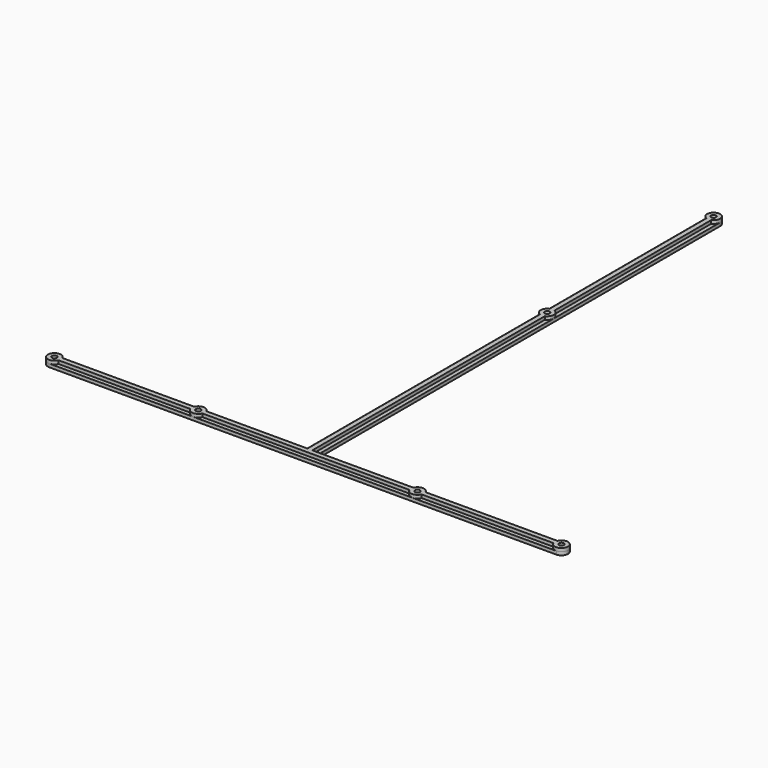
from build123d import *

# Parameters (mm, degrees)
F0_R     = 1.2192
F1_DEPTH = 1.5875
F2_R     = 3.17499
F3_R     = 1.2192
F4_DEPTH = 1.5875


# Not quite as in the source:
# - a fillet or chamfer is up to 0.001 mm smaller than in the source, because OpenCascade refuses the exact size


with BuildPart() as f1:
    # F0 (on Top) → F1 (new body)
    with BuildSketch(Plane.XY):
        Polygon((-127, 3.175), (-127, -3.175), (127, -3.175), (127, 3.175), (3.175, 3.175), (3.175, 250.825), (-3.175, 250.825), (-3.175, 3.175), align=None)
        with Locations((-123.825, 0)):
            Circle(F0_R, mode=Mode.SUBTRACT)
        with Locations((-53.5178, 0)):
            Circle(F0_R, mode=Mode.SUBTRACT)
        with Locations((53.5178, 0)):
            Circle(F0_R, mode=Mode.SUBTRACT)
        with Locations((123.825, 0)):
            Circle(F0_R, mode=Mode.SUBTRACT)
        with Locations((0, 146.05)):
            Circle(F0_R, mode=Mode.SUBTRACT)
        with Locations((0, 247.65)):
            Circle(F0_R, mode=Mode.SUBTRACT)
    extrude(amount=F1_DEPTH)

    # F2 (radius 3.175 in the source; OpenCascade refuses exactly that, so slightly less here)
    f2_edges = [f1.edges().sort_by_distance(p)[0] for p in [
        (-127, -3.175, 0.79375),
        (-127, 3.175, 0.79375),
        (127, 3.175, 0.79375),
        (127, -3.175, 0.79375),
        (-3.175, 250.825, 0.79375),
        (3.175, 250.825, 0.79375),
    ]]
    fillet(f2_edges, radius=F2_R)

    # F3 (on face) → F4 (join)
    with BuildSketch(Plane.XY.offset(1.5875)):
        with BuildLine():
            Line((-56.4611037746, 1.190625), (-120.8816962254, 1.190625))
            ThreePointArc((-120.8816962254, 1.190625), (-127, 0), (-120.8816962254, -1.190625))
            Line((-120.8816962254, -1.190625), (-56.4611037746, -1.190625))
            ThreePointArc((-56.4611037746, -1.190625), (-53.5178, -3.175), (-50.5744962254, -1.190625))
            Line((-50.5744962254, -1.190625), (50.5744962254, -1.190625))
            ThreePointArc((50.5744962254, -1.190625), (53.5178, -3.175), (56.4611037746, -1.190625))
            Line((56.4611037746, -1.190625), (120.8816962254, -1.190625))
            ThreePointArc((120.8816962254, -1.190625), (127, 0), (120.8816962254, 1.190625))
            Line((120.8816962254, 1.190625), (56.4611037746, 1.190625))
            ThreePointArc((56.4611037746, 1.190625), (53.5178, 3.175), (50.5744962254, 1.190625))
            Line((50.5744962254, 1.190625), (1.190625, 1.190625))
            Line((1.190625, 1.190625), (1.190625, 143.1066962254))
            ThreePointArc((1.190625, 143.1066962254), (3.175, 146.05), (1.190625, 148.9933037746))
            Line((1.190625, 148.9933037746), (1.190625, 244.7066962254))
            ThreePointArc((1.190625, 244.7066962254), (0, 250.825), (-1.190625, 244.7066962254))
            Line((-1.190625, 244.7066962254), (-1.190625, 148.9933037746))
            ThreePointArc((-1.190625, 148.9933037746), (-3.175, 146.05), (-1.190625, 143.1066962254))
            Line((-1.190625, 143.1066962254), (-1.190625, 1.190625))
            Line((-1.190625, 1.190625), (-50.5744962254, 1.190625))
            ThreePointArc((-50.5744962254, 1.190625), (-53.5178, 3.175), (-56.4611037746, 1.190625))
        make_face()
        with Locations((-123.825, 0)):
            Circle(F3_R, mode=Mode.SUBTRACT)
        with Locations((-53.5178, 0)):
            Circle(F3_R, mode=Mode.SUBTRACT)
        with Locations((53.5178, 0)):
            Circle(F3_R, mode=Mode.SUBTRACT)
        with Locations((123.825, 0)):
            Circle(F3_R, mode=Mode.SUBTRACT)
        with Locations((0, 146.05)):
            Circle(F3_R, mode=Mode.SUBTRACT)
        with Locations((0, 247.65)):
            Circle(F3_R, mode=Mode.SUBTRACT)
    extrude(amount=F4_DEPTH)


solid = f1.part
